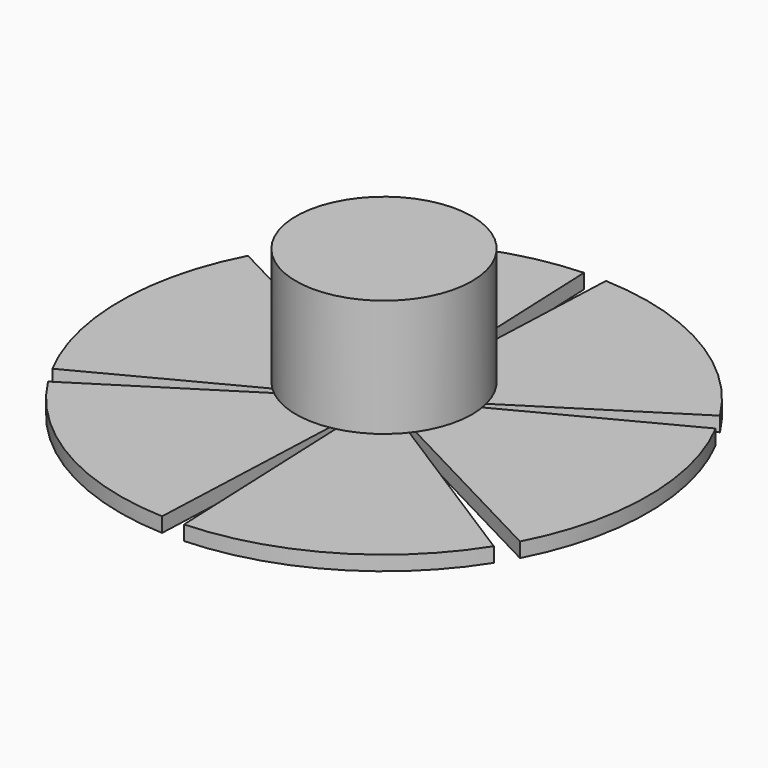
from build123d import *

# Parameters (mm, degrees)
F0_R            = 38.1
F1_DEPTH        = 50.8
F2_R            = 3.175
F3_DEPTH        = 6.35
F4_R            = 114.3
F5_DEPTH        = 6.35
F7_DEPTH        = 6.35
F7_COPIES_COUNT = 5
F7_COPIES_ANGLE = 240
F8_R            = 19.05
F9_DEPTH        = 6.35
F10_R           = 6.34999


# Not quite as in the source:
# - a fillet or chamfer is up to 0.001 mm smaller than in the source, because OpenCascade refuses the exact size
# - a pattern or mirror of a feature is missing from the dataset's text; its kind, count and spacing are read off the source's solid


with BuildPart() as f1:
    # F0 (on Top) → F1 (new body)
    with BuildSketch(Plane.XY):
        Circle(F0_R)
    extrude(amount=F1_DEPTH)

    # F2 (on face) → F3 (join)
    with BuildSketch(Plane(origin=(0, 0, 0), x_dir=(1, 0, 0), z_dir=(0, 0, -1))):
        Circle(F2_R)
    extrude(amount=F3_DEPTH)

    # F4 (on face) → F5 (join)
    with BuildSketch(Plane(origin=(0, 0, -6.35), x_dir=(1, 0, 0), z_dir=(0, 0, -1))):
        Circle(F4_R)
    extrude(amount=F5_DEPTH)

    # F6 (on face) → F7 (cut, through all)
    with BuildSketch(Plane(origin=(0, 0, -12.7), x_dir=(1, 0, 0), z_dir=(0, 0, -1))):
        with BuildLine():
            Line((16.880331728, 8.8293205148), (101.2819903679, 52.9759230889))
            ThreePointArc((101.2819903679, 52.9759230889), (98.9867036526, 57.15), (96.5194903679, 61.22481506))
            Line((96.5194903679, 61.22481506), (16.086581728, 10.2041358433))
            ThreePointArc((16.086581728, 10.2041358433), (16.4977839421, 9.525), (16.880331728, 8.8293205148))
        make_face()
        with BuildLine():
            ThreePointArc((96.5194903679, -61.22481506), (98.9867036526, -57.15), (101.2819903679, -52.9759230889))
            Line((101.2819903679, -52.9759230889), (16.880331728, -8.8293205148))
            ThreePointArc((16.880331728, -8.8293205148), (16.4977839421, -9.525), (16.086581728, -10.2041358433))
            Line((16.086581728, -10.2041358433), (96.5194903679, -61.22481506))
        make_face()
    f7 = extrude(amount=-F7_DEPTH, mode=Mode.SUBTRACT)

    # F7_copies: F7 ×5 about axis
    f7_copies_axis = Axis((0, 0, 0), (0, 0, 1))
    for i in range(1, F7_COPIES_COUNT):
        add(f7.rotate(f7_copies_axis, i * F7_COPIES_ANGLE / (F7_COPIES_COUNT - 1)), mode=Mode.SUBTRACT)

    # F8 (on face) → F9 (join)
    with BuildSketch(Plane(origin=(0, 0, -12.7), x_dir=(1, 0, 0), z_dir=(0, 0, -1))):
        Circle(F8_R)
    extrude(amount=F9_DEPTH)

    # F10 (radius 6.35 in the source; OpenCascade refuses exactly that, so slightly less here)
    f10_edges = [f1.edges().sort_by_distance(p)[0] for p in [
        (-19.05, 0, -19.05),
    ]]
    fillet(f10_edges, radius=F10_R)


solid = f1.part
